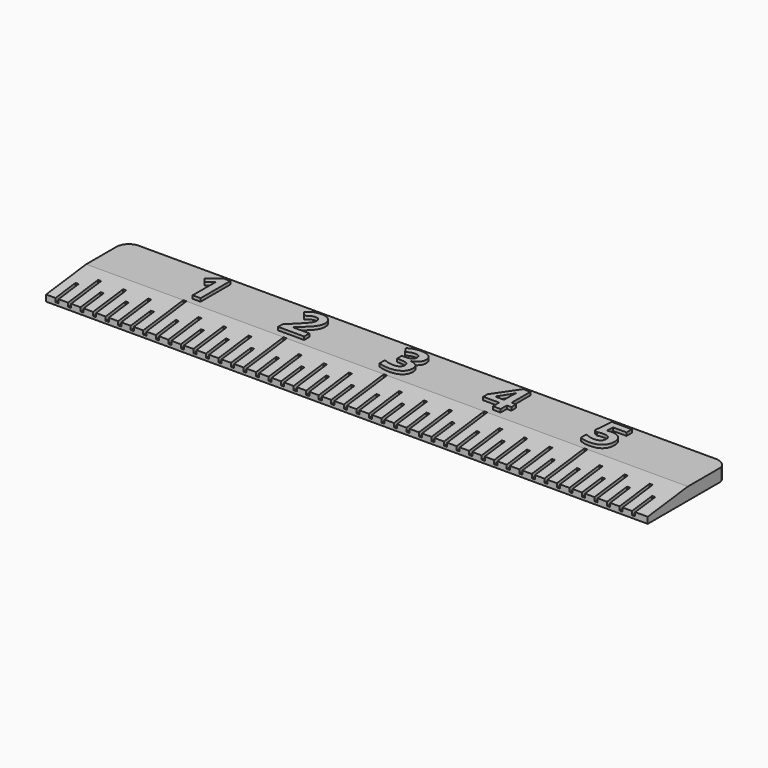
from build123d import *

# Parameters (mm, degrees)
F0_W         = 152.4
F0_H         = 25.4
F1_DEPTH     = 3.175
F2_W         = 0.79375
F2_H         = 12.7
F3_DEPTH     = 2.54
F4_W         = 0.79375
F4_H         = 9.525
F5_DEPTH     = 2.54
F6_W         = 0.79375
F6_H         = 6.35
F7_DEPTH     = 2.54
F8_TEXT_SIZE = 13.2291666667
F9_DEPTH     = 0.79375
F11_DEPTH    = 152.4010001
F13_DEPTH    = 25.4


# Not quite as in the source:
# - Text() gives the source's letters only with a copy of the font that has no kerning and outlines rounded to 1/6400 em; it was checked with that copy


with BuildPart() as f1:
    # F0 (on Top) → F1 (new body)
    with BuildSketch(Plane.XY):
        with Locations((-0.061262399, -5.0351110935)):
            Rectangle(F0_W, F0_H)
    extrude(amount=F1_DEPTH)

    # F2 (on face) → F3 (cut)
    with BuildSketch(Plane.XY.offset(3.175)):
        with Locations((-51.258137399, -11.3851110935)):
            Rectangle(F2_W, F2_H)
        with Locations((-25.858137399, -11.3851110935)):
            Rectangle(F2_W, F2_H)
        with Locations((-0.458137399, -11.3851110935)):
            Rectangle(F2_W, F2_H)
        with Locations((24.941862601, -11.3851110935)):
            Rectangle(F2_W, F2_H)
        with Locations((50.341862601, -11.3851110935)):
            Rectangle(F2_W, F2_H)
    extrude(amount=-F3_DEPTH, mode=Mode.SUBTRACT)

    # F4 (on face) → F5 (cut)
    with BuildSketch(Plane.XY.offset(3.175)):
        with Locations((-70.308137399, -12.9726110935)):
            Rectangle(F4_W, F4_H)
        with Locations((-63.958137399, -12.9726110935)):
            Rectangle(F4_W, F4_H)
        with Locations((-57.608137399, -12.9726110935)):
            Rectangle(F4_W, F4_H)
        with Locations((-32.208137399, -12.9726110935)):
            Rectangle(F4_W, F4_H)
        with Locations((-38.558137399, -12.9726110935)):
            Rectangle(F4_W, F4_H)
        with Locations((-44.908137399, -12.9726110935)):
            Rectangle(F4_W, F4_H)
        with Locations((-6.808137399, -12.9726110935)):
            Rectangle(F4_W, F4_H)
        with Locations((-13.158137399, -12.9726110935)):
            Rectangle(F4_W, F4_H)
        with Locations((-19.508137399, -12.9726110935)):
            Rectangle(F4_W, F4_H)
        with Locations((18.591862601, -12.9726110935)):
            Rectangle(F4_W, F4_H)
        with Locations((12.241862601, -12.9726110935)):
            Rectangle(F4_W, F4_H)
        with Locations((5.891862601, -12.9726110935)):
            Rectangle(F4_W, F4_H)
        with Locations((43.991862601, -12.9726110935)):
            Rectangle(F4_W, F4_H)
        with Locations((37.641862601, -12.9726110935)):
            Rectangle(F4_W, F4_H)
        with Locations((31.291862601, -12.9726110935)):
            Rectangle(F4_W, F4_H)
        with Locations((69.391862601, -12.9726110935)):
            Rectangle(F4_W, F4_H)
        with Locations((63.041862601, -12.9726110935)):
            Rectangle(F4_W, F4_H)
        with Locations((56.691862601, -12.9726110935)):
            Rectangle(F4_W, F4_H)
    extrude(amount=-F5_DEPTH, mode=Mode.SUBTRACT)

    # F6 (on face) → F7 (cut)
    with BuildSketch(Plane.XY.offset(3.175)):
        with Locations((-73.483137399, -14.5601110935)):
            Rectangle(F6_W, F6_H)
        with Locations((-67.133137399, -14.5601110935)):
            Rectangle(F6_W, F6_H)
        with Locations((-60.783137399, -14.5601110935)):
            Rectangle(F6_W, F6_H)
        with Locations((-54.433137399, -14.5601110935)):
            Rectangle(F6_W, F6_H)
        with Locations((-29.033137399, -14.5601110935)):
            Rectangle(F6_W, F6_H)
        with Locations((-35.383137399, -14.5601110935)):
            Rectangle(F6_W, F6_H)
        with Locations((-48.083137399, -14.5601110935)):
            Rectangle(F6_W, F6_H)
        with Locations((-41.733137399, -14.5601110935)):
            Rectangle(F6_W, F6_H)
        with Locations((-3.633137399, -14.5601110935)):
            Rectangle(F6_W, F6_H)
        with Locations((-9.983137399, -14.5601110935)):
            Rectangle(F6_W, F6_H)
        with Locations((-22.683137399, -14.5601110935)):
            Rectangle(F6_W, F6_H)
        with Locations((-16.333137399, -14.5601110935)):
            Rectangle(F6_W, F6_H)
        with Locations((21.766862601, -14.5601110935)):
            Rectangle(F6_W, F6_H)
        with Locations((15.416862601, -14.5601110935)):
            Rectangle(F6_W, F6_H)
        with Locations((2.716862601, -14.5601110935)):
            Rectangle(F6_W, F6_H)
        with Locations((9.066862601, -14.5601110935)):
            Rectangle(F6_W, F6_H)
        with Locations((47.166862601, -14.5601110935)):
            Rectangle(F6_W, F6_H)
        with Locations((40.816862601, -14.5601110935)):
            Rectangle(F6_W, F6_H)
        with Locations((28.116862601, -14.5601110935)):
            Rectangle(F6_W, F6_H)
        with Locations((34.466862601, -14.5601110935)):
            Rectangle(F6_W, F6_H)
        with Locations((72.566862601, -14.5601110935)):
            Rectangle(F6_W, F6_H)
        with Locations((66.216862601, -14.5601110935)):
            Rectangle(F6_W, F6_H)
        with Locations((53.516862601, -14.5601110935)):
            Rectangle(F6_W, F6_H)
        with Locations((59.866862601, -14.5601110935)):
            Rectangle(F6_W, F6_H)
    extrude(amount=-F7_DEPTH, mode=Mode.SUBTRACT)

    # F8 (on face) → F9 (join)
    with BuildSketch(Plane.XY.offset(3.175)):
        with Locations((-54.0228265266, -3.4476110935)):
            Text('1', F8_TEXT_SIZE, font='Open Sans', font_style=FontStyle.BOLD, text_align=(TextAlign.LEFT, TextAlign.BOTTOM))
        with Locations((-29.4558506151, -3.4476110935)):
            Text('2', F8_TEXT_SIZE, font='Open Sans', font_style=FontStyle.BOLD, text_align=(TextAlign.LEFT, TextAlign.BOTTOM))
        with Locations((-4.0103753547, -3.4476110935)):
            Text('3', F8_TEXT_SIZE, font='Open Sans', font_style=FontStyle.BOLD, text_align=(TextAlign.LEFT, TextAlign.BOTTOM))
        with Locations((21.2376959344, -3.4476110935)):
            Text('4', F8_TEXT_SIZE, font='Open Sans', font_style=FontStyle.BOLD, text_align=(TextAlign.LEFT, TextAlign.BOTTOM))
        with Locations((46.8309657911, -3.4476110935)):
            Text('5', F8_TEXT_SIZE, font='Open Sans', font_style=FontStyle.BOLD, text_align=(TextAlign.LEFT, TextAlign.BOTTOM))
    extrude(amount=F9_DEPTH)

    # F10 (on face) → F11 (cut, through all)
    with BuildSketch(Plane.YZ.offset(76.138737601)):
        Polygon((-17.7351110935, 3.175), (-17.7351110935, 1.5875), (-5.0351110935, 3.175), align=None)
    extrude(amount=-F11_DEPTH, mode=Mode.SUBTRACT)

    # F12 (on face) → F13 (cut)
    with BuildSketch(Plane.XY.offset(3.175)):
        with BuildLine():
            ThreePointArc((-76.261262399, 4.4898889065), (-75.3313264292, 6.7349529368), (-73.086262399, 7.6648889065))
            Line((-73.086262399, 7.6648889065), (-76.261262399, 7.6648889065))
            Line((-76.261262399, 7.6648889065), (-76.261262399, 4.4898889065))
        make_face()
        with BuildLine():
            ThreePointArc((73.086262399, 7.6648889065), (75.3313264292, 6.7349529368), (76.261262399, 4.4898889065))
            Line((76.261262399, 4.4898889065), (76.261262399, 7.6648889065))
            Line((76.261262399, 7.6648889065), (73.086262399, 7.6648889065))
        make_face()
    extrude(amount=-F13_DEPTH, mode=Mode.SUBTRACT)


solid = f1.part
